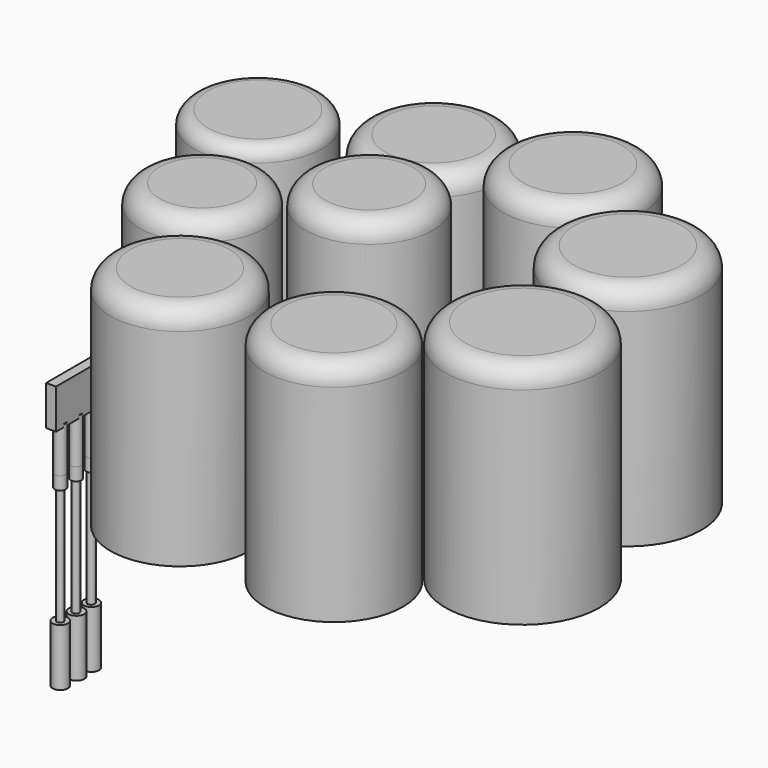
from build123d import *

# Parameters (mm, degrees)
F2_W           = 12.7
F2_H           = 76.2
F3_DEPTH       = 50.8
F4_R           = 5.8628476557
F5_DEPTH       = 6.35
F8_R           = 5.8441884283
F9_DEPTH       = 25.4
F10_R          = 3.4624203049
F11_DEPTH      = 35.56
F11_TAPER      = 3
F12_R          = 7.0320661699
F12_R_2        = 6.7211052485
F13_DEPTH      = 57.785
F13_DEPTH_BACK = 16.51
F14_R          = 4.4633349548
F14_R_2        = 4.5159221891
F14_R_3        = 4.641518377
F15_DEPTH      = 149.86
F16_R          = 9.8296366939
F16_R_2        = 9.9229407279
F16_R_3        = 9.6547726801
F17_DEPTH      = 73.025
F18_R          = 81.6235481259
F19_DEPTH      = 285.75
F20_R          = 17.78
F21_R          = 87.0621975567
F22_DEPTH      = 261.62
F23_R          = 89.1108416069
F24_DEPTH      = 289.56
F23_R_2        = 93.9746231805
F23_R_3        = 98.2513633913
F23_R_4        = 88.2596614963
F23_R_5        = 88.7911367864
F23_R_6        = 81.8118965518
F23_R_7        = 79.8119680434
F25_R          = 25.4
F25_2_R        = 25.4
F25_3_R        = 25.4
F25_4_R        = 25.4
F25_5_R        = 25.4
F25_6_R        = 25.4
F25_7_R        = 25.4
F25_8_R        = 25.4


# Not quite as in the source:
# - the program builds the solid bodies; features that only make, move or delete a surface that nothing else refers to are left out


with BuildPart() as f3:
    # F2 (on face) → F3 (new body)
    with BuildSketch(Plane(origin=(0, 0, 54.0316375996), x_dir=(1, 0, 0), z_dir=(0, 0, -1))):
        with Locations((-327.8094934464, 95.0275551417)):
            Rectangle(F2_W, F2_H)
    extrude(amount=-F3_DEPTH)

    # F4 (on face) → F5 (join)
    with BuildSketch(Plane(origin=(0, -56.9275551417, 0), x_dir=(-1, 0, 0), z_dir=(0, 1, 0))):
        with Locations((328.2679021358, 94.7593301535)):
            Circle(F4_R)
    extrude(amount=F5_DEPTH)

    # F6 (on face) → F7 (revolve)
    with BuildSketch(Plane(origin=(0, -50.5775551417, 0), x_dir=(-1, 0, 0), z_dir=(0, 1, 0))):
        with BuildLine():
            Line((333.9467644691, 100.5437831202), (329.2234577381, 100.5437831202))
            ThreePointArc((329.2234577381, 100.5437831202), (332.2283440821, 99.0822784788), (333.9467644691, 96.2165553361))
            Line((333.9467644691, 96.2165553361), (333.9467644691, 100.5437831202))
        make_face()
        with BuildLine():
            ThreePointArc((333.9467644691, 93.3021049708), (332.2283440821, 90.4363818281), (329.2234577381, 88.9748771867))
            Line((329.2234577381, 88.9748771867), (329.2234577381, 87.6910164952))
            Line((329.2234577381, 87.6910164952), (333.9467644691, 87.6910164952))
            Line((333.9467644691, 87.6910164952), (333.9467644691, 93.3021049708))
        make_face()
        with BuildLine():
            ThreePointArc((333.9467644691, 96.2165553361), (332.2283440821, 99.0822784788), (329.2234577381, 100.5437831202))
            Line((329.2234577381, 100.5437831202), (329.2234577381, 88.9748771867))
            ThreePointArc((329.2234577381, 88.9748771867), (332.2283440821, 90.4363818281), (333.9467644691, 93.3021049708))
            Line((333.9467644691, 93.3021049708), (333.9467644691, 96.2165553361))
        make_face()
    revolve(axis=Axis((-329.2234577381, -50.5775551417, 94.1173998077), (0, 0, -1)))

    # F8 (on face) → F9 (join)
    with BuildSketch(Plane.XY.offset(100.5437831202)):
        with Locations((-329.2234577381, -50.5775551417)):
            Circle(F8_R)
    extrude(amount=F9_DEPTH)

    # F10 (on face) → F11 (join)
    with BuildSketch(Plane.XY.offset(125.9437831202)):
        with Locations((-329.2234577381, -50.5775551417)):
            Circle(F10_R)
    extrude(amount=F11_DEPTH, taper=F11_TAPER)

    # F12 (on face) → F13 (join, two sides)
    with BuildSketch(Plane.XY) as f13_sk:
        with Locations((-327.7796208858, -118.4794306755)):
            Circle(F12_R)
        with Locations((-327.7796208858, -93.2544544339)):
            Circle(F12_R)
        with Locations((-327.7796208858, -69.1262111068)):
            Circle(F12_R_2)
    extrude(amount=F13_DEPTH)
    extrude(f13_sk.sketch, amount=-F13_DEPTH_BACK)

    # F14 (on face) → F15 (join)
    with BuildSketch(Plane(origin=(0, 0, -16.51), x_dir=(1, 0, 0), z_dir=(0, 0, -1))):
        with Locations((-327.7796208858, 118.4794306755)):
            Circle(F14_R)
        with Locations((-327.7796208858, 93.3841094375)):
            Circle(F14_R_2)
        with Locations((-327.9483318329, 68.9324364066)):
            Circle(F14_R_3)
    extrude(amount=F15_DEPTH)

    # F16 (on face) → F17 (join)
    with BuildSketch(Plane(origin=(0, 0, -166.37), x_dir=(1, 0, 0), z_dir=(0, 0, -1))):
        with Locations((-327.7796208858, 118.4794306755)):
            Circle(F16_R)
        with Locations((-327.7796208858, 92.5656706095)):
            Circle(F16_R_2)
        with Locations((-327.7796208858, 68.6676949263)):
            Circle(F16_R_3)
    extrude(amount=F17_DEPTH)


with BuildPart() as f19:
    # F18 (on face) → F19 (new body)
    with BuildSketch(Plane(origin=(0, 0, 54.0316375996), x_dir=(1, 0, 0), z_dir=(0, 0, -1))):
        with Locations((-256.3232183456, -107.8240275383)):
            Circle(F18_R)
    extrude(amount=-F19_DEPTH)

    # F20
    f20_edges = [f19.edges().sort_by_distance(p)[0] for p in [
        (-337.946766, 107.824028, 339.781638),
    ]]
    fillet(f20_edges, radius=F20_R)


with BuildPart() as f22:
    # F21 (on face) → F22 (new body)
    with BuildSketch(Plane(origin=(0, 0, 54.0316375996), x_dir=(1, 0, 0), z_dir=(0, 0, -1))):
        with Locations((-114.6806776524, -211.5678787231)):
            Circle(F21_R)
    extrude(amount=-F22_DEPTH)

    # F25
    f25_edges = [f22.edges().sort_by_distance(p)[0] for p in [
        (-201.742875, 211.567879, 315.651638),
    ]]
    fillet(f25_edges, radius=F25_R)


with BuildPart() as f24:
    # F23 (on face) → F24 (new body)
    with BuildSketch(Plane(origin=(0, 0, 54.0316375996), x_dir=(1, 0, 0), z_dir=(0, 0, -1))):
        with Locations((67.6698461175, -206.0038298368)):
            Circle(F23_R)
    extrude(amount=-F24_DEPTH)

    # F25#2
    f25_2_edges = [f24.edges().sort_by_distance(p)[0] for p in [
        (-21.440995, 206.00383, 343.591638),
    ]]
    fillet(f25_2_edges, radius=F25_2_R)


with BuildPart() as f24b:
    # F23 (on face) → F24, piece 2 (new body)
    with BuildSketch(Plane(origin=(0, 0, 54.0316375996), x_dir=(1, 0, 0), z_dir=(0, 0, -1))):
        with Locations((220.1114147902, -103.2785326242)):
            Circle(F23_R_2)
    extrude(amount=-F24_DEPTH)

    # F25#3
    f25_3_edges = [f24b.edges().sort_by_distance(p)[0] for p in [
        (126.136792, 103.278533, 343.591638),
    ]]
    fillet(f25_3_edges, radius=F25_3_R)


with BuildPart() as f24c:
    # F23 (on face) → F24, piece 3 (new body)
    with BuildSketch(Plane(origin=(0, 0, 54.0316375996), x_dir=(1, 0, 0), z_dir=(0, 0, -1))):
        with Locations((241.139113903, 91.3788825274)):
            Circle(F23_R_3)
    extrude(amount=-F24_DEPTH)

    # F25#4
    f25_4_edges = [f24c.edges().sort_by_distance(p)[0] for p in [
        (142.887751, -91.378883, 343.591638),
    ]]
    fillet(f25_4_edges, radius=F25_4_R)


with BuildPart() as f24d:
    # F23 (on face) → F24, piece 4 (new body)
    with BuildSketch(Plane(origin=(0, 0, 54.0316375996), x_dir=(1, 0, 0), z_dir=(0, 0, -1))):
        with Locations((96.867673099, 212.2096270323)):
            Circle(F23_R_4)
    extrude(amount=-F24_DEPTH)

    # F25#5
    f25_5_edges = [f24d.edges().sort_by_distance(p)[0] for p in [
        (8.608012, -212.209627, 343.591638),
    ]]
    fillet(f25_5_edges, radius=F25_5_R)


with BuildPart() as f24e:
    # F23 (on face) → F24, piece 5 (new body)
    with BuildSketch(Plane(origin=(0, 0, 54.0316375996), x_dir=(1, 0, 0), z_dir=(0, 0, -1))):
        with Locations((-98.6495241523, 213.7624174356)):
            Circle(F23_R_5)
    extrude(amount=-F24_DEPTH)

    # F25#6
    f25_6_edges = [f24e.edges().sort_by_distance(p)[0] for p in [
        (-187.440661, -213.762417, 343.591638),
    ]]
    fillet(f25_6_edges, radius=F25_6_R)


with BuildPart() as f24f:
    # F23 (on face) → F24, piece 6 (new body)
    with BuildSketch(Plane(origin=(0, 0, 54.0316375996), x_dir=(1, 0, 0), z_dir=(0, 0, -1))):
        with Locations((-64.5457431674, -45.8989851177)):
            Circle(F23_R_6)
    extrude(amount=-F24_DEPTH)

    # F25#7
    f25_7_edges = [f24f.edges().sort_by_distance(p)[0] for p in [
        (-146.35764, 45.898985, 343.591638),
    ]]
    fillet(f25_7_edges, radius=F25_7_R)


with BuildPart() as f24g:
    # F23 (on face) → F24, piece 7 (new body)
    with BuildSketch(Plane(origin=(0, 0, 54.0316375996), x_dir=(1, 0, 0), z_dir=(0, 0, -1))):
        with Locations((-196.1999088526, 56.3914589584)):
            Circle(F23_R_7)
    extrude(amount=-F24_DEPTH)

    # F25#8
    f25_8_edges = [f24g.edges().sort_by_distance(p)[0] for p in [
        (-276.011877, -56.391459, 343.591638),
    ]]
    fillet(f25_8_edges, radius=F25_8_R)


solid = Compound([f3.part, f19.part, f22.part, f24.part, f24b.part, f24c.part, f24d.part, f24e.part, f24f.part, f24g.part])
